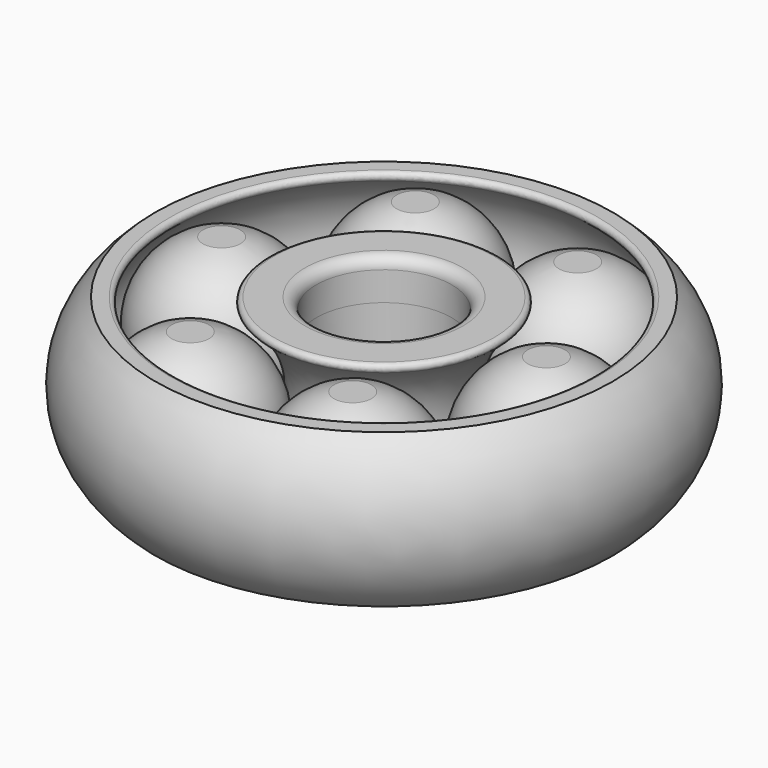
from build123d import *

# Parameters (mm, degrees)
F6_COUNT  = 6
F7_R      = 1.016
F7_2_R    = 1.016
F8_R      = 21.6007665794
F8_R_2    = 15.24
F11_R     = 2.54
F12_R     = 15.24
F13_DEPTH = 38.354


# Not quite as in the source:
# - a feature names something its author has since deleted; it is built from what else it names


with BuildPart() as f2:
    # F0 (on Front) → F2 (revolve)
    with BuildSketch(Plane.XZ):
        with BuildLine():
            ThreePointArc((21.6007665794, 17.272), (13.716, 0), (21.6007665794, -17.272))
            Line((21.6007665794, -17.272), (28.5397996541, -17.272))
            ThreePointArc((28.5397996541, -17.272), (17.526, 0), (28.5397996541, 17.272))
            Line((28.5397996541, 17.272), (21.6007665794, 17.272))
        make_face()
    revolve(axis=Axis((0, 0, -3.9324210957), (0, 0, -1)))

    # F7#2
    f7_2_edges = [f2.edges().sort_by_distance(p)[0] for p in [
        (-28.5398, 0, 17.272),
        (-28.5398, 0, -17.272),
    ]]
    fillet(f7_2_edges, radius=F7_2_R)

    # F8 (on face) → F9 (join, up to the next surface of F2)
    with BuildSketch(Plane(origin=(0, 0, -17.272), x_dir=(1, 0, 0), z_dir=(0, 0, -1))):
        Circle(F8_R)
        Circle(F8_R_2, mode=Mode.SUBTRACT)
    extrude(until=Until.NEXT, dir=(0, 0, 1))

    # F10: F2 across plane


with BuildPart() as f3:
    # F0 (on Front) → F3 (revolve)
    with BuildSketch(Plane.XZ):
        with BuildLine():
            ThreePointArc((44.6122003459, 17.272), (55.626, 0), (44.6122003459, -17.272))
            Line((44.6122003459, -17.272), (51.5512334206, -17.272))
            ThreePointArc((51.5512334206, -17.272), (59.436, 0), (51.5512334206, 17.272))
            Line((51.5512334206, 17.272), (44.6122003459, 17.272))
        make_face()
    revolve(axis=Axis((0, 0, -3.9324210957), (0, 0, -1)))

    # F7
    f7_edges = [f3.edges().sort_by_distance(p)[0] for p in [
        (-44.6122, 0, 17.272),
        (-44.6122, 0, -17.272),
    ]]
    fillet(f7_edges, radius=F7_R)


with BuildPart() as f5:
    # F4 (on Front) → F5 (revolve)
    with BuildSketch(Plane.XZ):
        with BuildLine():
            Line((36.576, -17.272), (36.576, 17.272))
            Line((36.576, 17.272), (32.3562350776, 17.272))
            ThreePointArc((32.3562350776, 17.272), (18.796, 0), (32.3562350776, -17.272))
            Line((32.3562350776, -17.272), (36.576, -17.272))
        make_face()
    revolve(axis=Axis((36.576, 0, 0), (0, 0, -1)))


with BuildPart() as f6_1:
    # F6: instance of F5
    add(f5.part.rotate(Axis((0, 0, -3.9324210957), (0, 0, -1)), 1 * 360 / F6_COUNT))


with BuildPart() as f6_2:
    # F6: instance of F5
    add(f5.part.rotate(Axis((0, 0, -3.9324210957), (0, 0, -1)), 2 * 360 / F6_COUNT))


with BuildPart() as f6_3:
    # F6: instance of F5
    add(f5.part.rotate(Axis((0, 0, -3.9324210957), (0, 0, -1)), 3 * 360 / F6_COUNT))


with BuildPart() as f6_4:
    # F6: instance of F5
    add(f5.part.rotate(Axis((0, 0, -3.9324210957), (0, 0, -1)), 4 * 360 / F6_COUNT))


with BuildPart() as f6_5:
    # F6: instance of F5
    add(f5.part.rotate(Axis((0, 0, -3.9324210957), (0, 0, -1)), 5 * 360 / F6_COUNT))


with BuildPart() as f2_1:
    add(f2.part)
    add(f2.part.mirror(Plane.XY))

    # F11
    f11_edges = [f2_1.edges().sort_by_distance(p)[0] for p in [
        (-15.24, 0, -17.272),
        (-15.24, 0, 17.272),
    ]]
    fillet(f11_edges, radius=F11_R)

    # F12 (on face) → F13 (cut)
    with BuildSketch(Plane(origin=(0, 0, -17.272), x_dir=(1, 0, 0), z_dir=(0, 0, -1))):
        Circle(F12_R)
    extrude(amount=-F13_DEPTH, mode=Mode.SUBTRACT)


solid = Compound([f3.part, f5.part, f6_1.part, f6_2.part, f6_3.part, f6_4.part, f6_5.part, f2_1.part])
